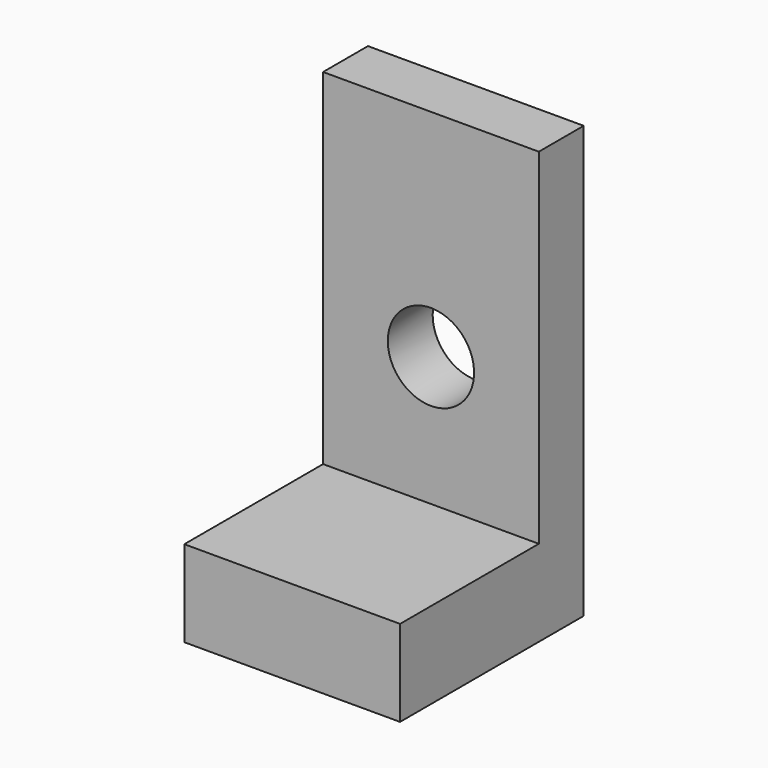
from build123d import *

# Parameters (mm, degrees)
F0_W     = 50
F0_H     = 100
F1_DEPTH = 13
F2_W     = 50
F2_H     = 20
F3_DEPTH = 40.2
F4_R     = 10
F5_DEPTH = 66.4


# Not quite as in the source:
# - a feature names something its author has since deleted; it is built from what else it names


with BuildPart() as f1:
    # F0 (on Front) → F1 (new body)
    with BuildSketch(Plane.XZ):
        Rectangle(F0_W, F0_H)
    extrude(amount=F1_DEPTH)

    # F2 (on face) → F3 (join)
    with BuildSketch(Plane.XZ.offset(13)):
        with Locations((0, -40)):
            Rectangle(F2_W, F2_H)
    extrude(amount=F3_DEPTH)

    # F4 (on face) → F5 (cut)
    with BuildSketch(Plane(origin=(0, 0, 0), x_dir=(-1, 0, 0), z_dir=(0, 1, 0))):
        Circle(F4_R)
    extrude(amount=-F5_DEPTH, mode=Mode.SUBTRACT)


solid = f1.part
